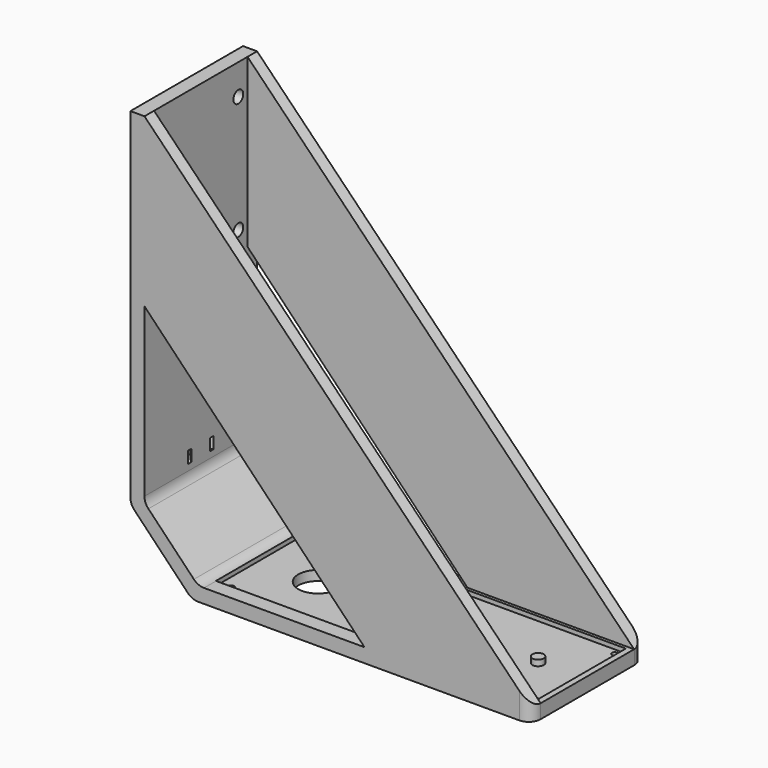
from build123d import *

# Parameters (mm, degrees)
F1_DEPTH     = 60
F2_W         = 137
F2_H         = 47.15
F3_DEPTH     = 1.85
F5_D         = 2.5
F5_DEPTH     = 3
F5_TIP       = 0.7510757738
F4_R         = 2.425
F6_DEPTH     = 2.5
F8_D         = 5.25
F9_T1_DEPTH  = 60
F9_T6_DEPTH  = 60
F9_T12_DEPTH = 60
F9_T18_DEPTH = 60
F9_T25_DEPTH = 60
F9_T31_DEPTH = 60
F9_T34_DEPTH = 72.0912564168
F9_T36_DEPTH = 72.7642259517
F4_R_2       = 8.5
F4_R_3       = 7.5
F10_DEPTH    = 25
F12_DEPTH    = 5.1
F14_DEPTH    = 5.1
F15_R        = 5
F18_DEPTH    = 2.5
F21_DEPTH    = 2.5


# Not quite as in the source:
# - a fillet or chamfer that OpenCascade refuses, or shapes differently, is made with other operations: its cross-section is extruded or revolved along the edge and cut away or added
# - a feature names something its author has since deleted; it is built from what else it names


with BuildPart() as f1:
    # F0 (on Front) → F1 (new body)
    with BuildSketch(Plane.XZ):
        Polygon((-22.8349631621, 174.7265526258), (-28.8349631621, 174.7265526258), (-28.8349631621, 29.7265526258), (-28.8349631621, 27.3083013424), (-2.5528451903, 0), (0, 0), (141.95, 0), (141.95, 6), (0, 6), (-22.8349631621, 29.7265526258), (-22.8349631621, 151.506786451), align=None)
    extrude(amount=F1_DEPTH)

    # F2 (on face) → F3 (cut)
    with BuildSketch(Plane.XY.offset(6)):
        with Locations((70.975, -30)):
            Rectangle(F2_W, F2_H)
    extrude(amount=-F3_DEPTH, mode=Mode.SUBTRACT)

    # F5
    with Locations(Plane.XY.offset(4.15)):
        with Locations((7.025, -8.9), (136.825, -8.9), (136.825, -51.1), (7.025, -51.1)):
            Hole(F5_D / 2, depth=F5_DEPTH)
            with Locations((0, 0, -(F5_DEPTH + F5_TIP / 2))):  # 118° drill point
                Cone(0, F5_D / 2, F5_TIP, mode=Mode.SUBTRACT)

    # F4 (on face) → F6 (join)
    with BuildSketch(Plane.XY.offset(4.15)):
        with Locations((40.225, -30)):
            Circle(F4_R)
        with Locations((120.925, -30)):
            Circle(F4_R)
    extrude(amount=F6_DEPTH)

    # F8 (through all)
    with Locations(Plane.YZ.offset(-22.8349631621)):
        with Locations((-50, 161.7265526258), (-10, 161.7265526258), (-10, 111.7265526258), (-50, 111.7265526258)):
            Hole(F8_D / 2)

    # F9: fillet of radius 6 on 4 edges, made by hand

    # F9_s2 → F9_t1 (join)
    with BuildSketch(Plane.XZ):
        with BuildLine():
            ThreePointArc((-22.8349631621, 32.1448039092), (-22.3999669258, 29.9018743269), (-21.1580521252, 27.9841667203))
            Line((-21.1580521252, 27.9841667203), (-22.8349631621, 29.7265526258))
            Line((-22.8349631621, 29.7265526258), (-22.8349631621, 32.1448039092))
        make_face()
    extrude(amount=F9_T1_DEPTH)


with BuildPart() as f9_tool4:
    # F9_s5 → F9_t6 (new body)
    with BuildSketch(Plane.XZ):
        with BuildLine():
            ThreePointArc((-1.7702437727, 7.8393628111), (0.2037840091, 6.4789573841), (2.5528451903, 6))
            Line((2.5528451903, 6), (0, 6))
            Line((0, 6), (-1.7702437727, 7.8393628111))
        make_face()
    extrude(amount=F9_T6_DEPTH)

    split(bisect_by=Plane.YZ.offset(2.475), keep=Keep.BOTTOM)

    split(bisect_by=Plane.XZ.offset(6.425), keep=Keep.BOTTOM)


with BuildPart() as f1_1:
    add(f1.part)

    # F9_t3: union F9_tool4
    add(f9_tool4.part)


with BuildPart() as f9_tool10:
    # F9_s11 → F9_t12 (new body)
    with BuildSketch(Plane.XZ):
        with BuildLine():
            ThreePointArc((-1.7702437727, 7.8393628111), (0.2037840091, 6.4789573841), (2.5528451903, 6))
            Line((2.5528451903, 6), (0, 6))
            Line((0, 6), (-1.7702437727, 7.8393628111))
        make_face()
    extrude(amount=F9_T12_DEPTH)

    split(bisect_by=Plane.YZ.offset(2.475), keep=Keep.TOP)

    split(bisect_by=Plane.XZ.offset(6.425), keep=Keep.BOTTOM)


with BuildPart() as f1_2:
    add(f1_1.part)

    # F9_t9: union F9_tool10
    add(f9_tool10.part)


with BuildPart() as f9_tool16:
    # F9_s17 → F9_t18 (new body)
    with BuildSketch(Plane.XZ):
        with BuildLine():
            ThreePointArc((-1.7702437727, 7.8393628111), (0.2037840091, 6.4789573841), (2.5528451903, 6))
            Line((2.5528451903, 6), (0, 6))
            Line((0, 6), (-1.7702437727, 7.8393628111))
        make_face()
    extrude(amount=F9_T18_DEPTH)

    split(bisect_by=Plane.XZ.offset(53.575), keep=Keep.BOTTOM)

    split(bisect_by=Plane.YZ.offset(2.475), keep=Keep.BOTTOM)

    split(bisect_by=Plane.XZ.offset(6.425), keep=Keep.TOP)


with BuildPart() as f1_3:
    add(f1_2.part)

    # F9_t15: union F9_tool16
    add(f9_tool16.part)


with BuildPart() as f9_tool23:
    # F9_s24 → F9_t25 (new body)
    with BuildSketch(Plane.XZ):
        with BuildLine():
            ThreePointArc((-1.7702437727, 7.8393628111), (0.2037840091, 6.4789573841), (2.5528451903, 6))
            Line((2.5528451903, 6), (0, 6))
            Line((0, 6), (-1.7702437727, 7.8393628111))
        make_face()
    extrude(amount=F9_T25_DEPTH)

    split(bisect_by=Plane.XZ.offset(53.575), keep=Keep.TOP)

    split(bisect_by=Plane.YZ.offset(2.475), keep=Keep.BOTTOM)


with BuildPart() as f1_4:
    add(f1_3.part)

    # F9_t22: union F9_tool23
    add(f9_tool23.part)


with BuildPart() as f9_tool29:
    # F9_s30 → F9_t31 (new body)
    with BuildSketch(Plane.XZ):
        with BuildLine():
            ThreePointArc((-1.7702437727, 7.8393628111), (0.2037840091, 6.4789573841), (2.5528451903, 6))
            Line((2.5528451903, 6), (0, 6))
            Line((0, 6), (-1.7702437727, 7.8393628111))
        make_face()
    extrude(amount=F9_T31_DEPTH)

    split(bisect_by=Plane.XZ.offset(53.575), keep=Keep.TOP)

    split(bisect_by=Plane.YZ.offset(2.475), keep=Keep.TOP)


with BuildPart() as f1_5:
    add(f1_4.part)

    # F9_t28: union F9_tool29
    add(f9_tool29.part)

    # F9_s35 → F9_t34 (cut)
    with BuildSketch(Plane.XZ.offset(-6.0456282084)):
        with BuildLine():
            ThreePointArc((-27.1580521252, 25.5659154369), (-28.3999669258, 27.4836230436), (-28.8349631621, 29.7265526258))
            Line((-28.8349631621, 29.7265526258), (-28.8349631621, 27.3083013424))
            Line((-28.8349631621, 27.3083013424), (-27.1580521252, 25.5659154369))
        make_face()
    extrude(amount=F9_T34_DEPTH, mode=Mode.SUBTRACT)

    # F9_s37 → F9_t36 (cut)
    with BuildSketch(Plane.XZ.offset(-6.3821129759)):
        with BuildLine():
            ThreePointArc((0, 0), (-2.3490611813, 0.4789573841), (-4.3230889631, 1.8393628111))
            Line((-4.3230889631, 1.8393628111), (-2.5528451903, 0))
            Line((-2.5528451903, 0), (0, 0))
        make_face()
    extrude(amount=F9_T36_DEPTH, mode=Mode.SUBTRACT)

    # F4 (on face) → F10 (cut)
    with BuildSketch(Plane.XY.offset(4.15)):
        with Locations((27.225, -30)):
            Circle(F4_R_2)
        with Locations((92.925, -30)):
            Circle(F4_R_3)
    extrude(amount=-F10_DEPTH, mode=Mode.SUBTRACT)

    # F11 (on face) → F12 (join)
    with BuildSketch(Plane(origin=(0, 0, 0), x_dir=(-1, 0, 0), z_dir=(0, 1, 0))):
        Polygon((22.8349631621, 103.4356782675), (22.8349631621, 174.7265526258), (-141.95, 6), (-70.9393056499, 6), align=None)
    extrude(amount=-F12_DEPTH)

    # F13 (on face) → F14 (join)
    with BuildSketch(Plane.XZ.offset(60)):
        Polygon((141.95, 6), (-22.8349631621, 174.7265526258), (-22.8349631621, 103.4356782675), (70.9393056499, 6), align=None)
    extrude(amount=-F14_DEPTH)

    # F15
    f15_edges = [f1_5.edges().sort_by_distance(p)[0] for p in [
        (141.95, -60, 3),
        (141.95, 0, 3),
    ]]
    fillet(f15_edges, radius=F15_R)

    # F17 (on line) → F18 (cut, symmetric)
    with BuildSketch(Plane.XY.offset(94.7265526258)):
        with BuildLine():
            Line((-21.5895338884, -23.119), (-22.8349631621, -23.119))
            ThreePointArc((-22.8349631621, -23.119), (-26.8349631621, -29.9997827216), (-22.8349631621, -36.8805654433))
            Line((-22.8349631621, -36.8805654433), (-21.7005347336, -36.8805654433))
            Line((-21.7005347336, -36.8805654433), (-21.7005347336, -34.9997827216))
            Line((-21.7005347336, -34.9997827216), (-22.8349631621, -34.9997827216))
            ThreePointArc((-22.8349631621, -34.9997827216), (-25.2691290512, -29.9997827216), (-22.8349631621, -24.9997827216))
            Line((-22.8349631621, -24.9997827216), (-21.5895338884, -24.9997827216))
            Line((-21.5895338884, -24.9997827216), (-21.5895338884, -23.119))
        make_face()
    extrude(amount=F18_DEPTH, both=True, mode=Mode.SUBTRACT)

    # F20 (on offset) → F21 (cut, symmetric)
    with BuildSketch(Plane.XY.offset(37.3265526258)):
        with BuildLine():
            Line((-21.657592603, -23.1192172784), (-22.9030218767, -23.1192172784))
            ThreePointArc((-22.9030218767, -23.1192172784), (-26.9030218767, -30), (-22.9030218767, -36.8807827216))
            Line((-22.9030218767, -36.8807827216), (-21.7685934482, -36.8807827216))
            Line((-21.7685934482, -36.8807827216), (-21.7685934482, -35))
            Line((-21.7685934482, -35), (-22.9030218767, -35))
            ThreePointArc((-22.9030218767, -35), (-25.3371877657, -30), (-22.9030218767, -25))
            Line((-22.9030218767, -25), (-21.657592603, -25))
            Line((-21.657592603, -25), (-21.657592603, -23.1192172784))
        make_face()
    extrude(amount=F21_DEPTH, both=True, mode=Mode.SUBTRACT)


solid = f1_5.part
